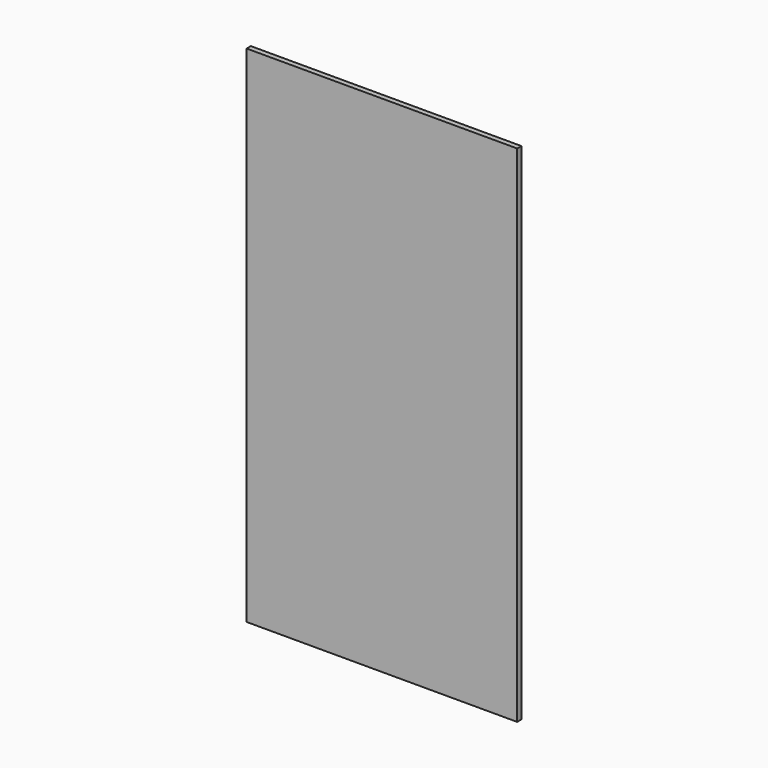
from build123d import *

# Parameters (mm, degrees)
F0_W         = 82
F0_H         = 153
F1_DEPTH     = 1.6
F2_TEXT_SIZE = 34.7222222222
F3_DEPTH     = 0.8


# Not quite as in the source:
# - Text() gives the source's letters only with a copy of the font that has no kerning and outlines rounded to 1/6400 em; it was checked with that copy


with BuildPart() as f1:
    # F0 (on Front) → F1 (new body)
    with BuildSketch(Plane.XZ):
        with Locations((-41, 0)):
            Rectangle(F0_W, F0_H)
    extrude(amount=F1_DEPTH)

    # F2 (on face) → F3 (cut)
    with BuildSketch(Plane(origin=(0, 0, 0), x_dir=(-1, 0, 0), z_dir=(0, 1, 0))):
        with Locations(Location((42, 49.4466145833), (0, 0, -90))):
            Text('ORCA', F2_TEXT_SIZE, font='Open Sans', font_style=FontStyle.BOLD, text_align=(TextAlign.LEFT, TextAlign.BOTTOM))
    extrude(amount=-F3_DEPTH, mode=Mode.SUBTRACT)


solid = f1.part
